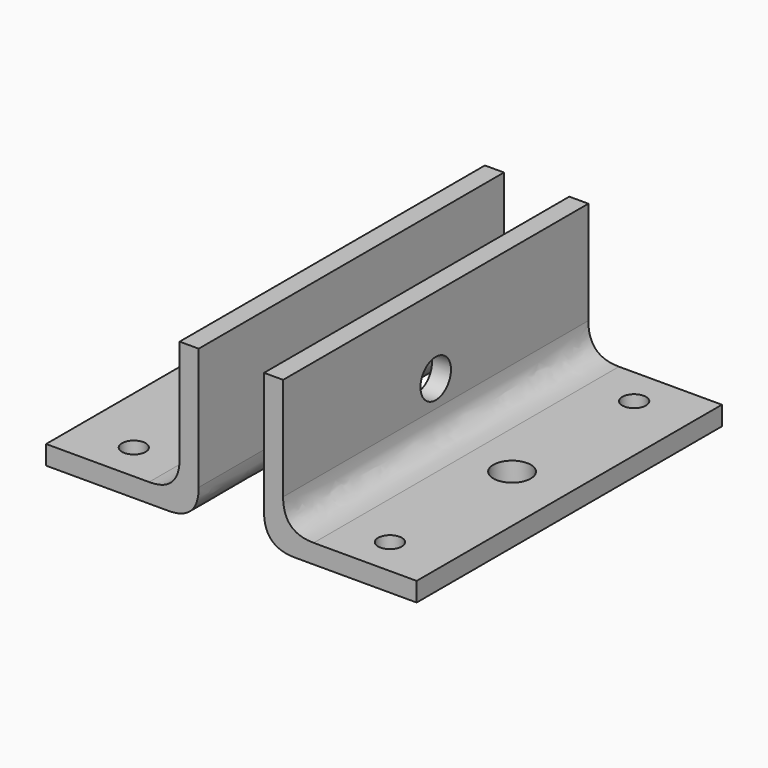
from build123d import *

# Parameters (mm, degrees)
F0_W           = 25.4
F0_H           = 63.5
F1_DEPTH       = 3.175
F2_W           = 3.175
F2_H           = 63.5
F3_DEPTH       = 22.225
F4_R           = 3.175
F5_DEPTH       = 3.175
F6_R           = 1.9685
F7_DEPTH       = 3.175
F8_R           = 1.9685
F9_DEPTH       = 3.175
F10_R          = 3.1115
F11_DEPTH      = 3.175
F12_W          = 25.4
F12_H          = 63.5
F13_DEPTH      = 3.175
F14_R          = 3.1115
F15_R          = 1.9685
F16_DEPTH      = 3.175
F17_W          = 3.175
F17_H          = 63.5
F18_DEPTH      = 22.225
F19_R          = 3.175
F20_DEPTH      = 3.175
F21_T1_DEPTH   = 63.5
F21_T3_DEPTH   = 88.9
F21_2_T1_DEPTH = 63.5
F21_2_T3_DEPTH = 88.9


# Not quite as in the source:
# - a fillet or chamfer that OpenCascade refuses, or shapes differently, is made with other operations: its cross-section is extruded or revolved along the edge and cut away or added


with BuildPart() as f1:
    # F0 (on Top) → F1 (new body)
    with BuildSketch(Plane.XY):
        with Locations((-29.1409659298, -4.4768862426)):
            Rectangle(F0_W, F0_H)
    extrude(amount=F1_DEPTH)

    # F2 (on face) → F3 (join)
    with BuildSketch(Plane.XY.offset(3.175)):
        with Locations((-18.0284659298, -4.4768862426)):
            Rectangle(F2_W, F2_H)
    extrude(amount=F3_DEPTH)

    # F4 (on face) → F5 (cut)
    with BuildSketch(Plane(origin=(-19.6159659298, 0, 0), x_dir=(0, -1, 0), z_dir=(-1, 0, 0))):
        with Locations((4.4768862426, 12.7)):
            Circle(F4_R)
    extrude(amount=-F5_DEPTH, mode=Mode.SUBTRACT)

    # F6 (on face) → F7 (cut)
    with BuildSketch(Plane.XY.offset(3.175)):
        with Locations((-32.3159659298, 20.9231137574)):
            Circle(F6_R)
    extrude(amount=-F7_DEPTH, mode=Mode.SUBTRACT)

    # F8 (on face) → F9 (cut)
    with BuildSketch(Plane.XY.offset(3.175)):
        with Locations((-32.3159659298, -29.8768862426)):
            Circle(F8_R)
    extrude(amount=-F9_DEPTH, mode=Mode.SUBTRACT)

    # F10 (on face) → F11 (cut)
    with BuildSketch(Plane.XY.offset(3.175)):
        with Locations((-32.3159659298, -4.4768862426)):
            Circle(F10_R)
    extrude(amount=-F11_DEPTH, mode=Mode.SUBTRACT)

    # F21: fillet of radius 5.08 on 2 edges, made by hand

    # F21_s2 → F21_t1 (join)
    with BuildSketch(Plane.XZ.offset(-27.2731137574)):
        with BuildLine():
            add(Edge.make_bspline(
                [(-19.6159659298, 8.255), (-19.6159659298, 3.175), (-24.6959659298, 3.175)],
                knots=[0, 0, 0, 1, 1, 1], degree=2, weights=[1, 1, 1]))
            Line((-24.6959659298, 3.175), (-19.6159659298, 3.175))
            Line((-19.6159659298, 3.175), (-19.6159659298, 8.255))
        make_face()
    extrude(amount=F21_T1_DEPTH)

    # F21_s4 → F21_t3 (cut)
    with BuildSketch(Plane.XZ.offset(-39.9731137574)):
        with BuildLine():
            add(Edge.make_bspline(
                [(-16.4409659298, 5.08), (-16.4409659298, 0), (-21.5209659298, 0)],
                knots=[0, 0, 0, 1, 1, 1], degree=2, weights=[1, 1, 1]))
            Line((-21.5209659298, 0), (-16.4409659298, 0))
            Line((-16.4409659298, 0), (-16.4409659298, 5.08))
        make_face()
    extrude(amount=F21_T3_DEPTH, mode=Mode.SUBTRACT)


with BuildPart() as f13:
    # F12 (on Top) → F13 (new body)
    with BuildSketch(Plane.XY):
        with Locations((7.1329429418, -4.4768862426)):
            Rectangle(F12_W, F12_H)
    extrude(amount=F13_DEPTH)

    # F14 (on face) + F15 (on face) → F16 (cut)
    with BuildSketch(Plane.XY.offset(3.175)):
        with Locations((10.3079429418, -4.4768862426)):
            Circle(F14_R)
    with BuildSketch(Plane.XY.offset(3.175)):
        with Locations((10.3079429418, 20.9231137574)):
            Circle(F15_R)
        with Locations((10.3079429418, -29.8768862426)):
            Circle(F15_R)
    extrude(amount=-F16_DEPTH, mode=Mode.SUBTRACT)

    # F17 (on face) → F18 (join)
    with BuildSketch(Plane.XY.offset(3.175)):
        with Locations((-3.9795570582, -4.4768862426)):
            Rectangle(F17_W, F17_H)
    extrude(amount=F18_DEPTH)

    # F19 (on face) → F20 (cut)
    with BuildSketch(Plane.YZ.offset(-2.3920570582)):
        with Locations((-4.4768862426, 12.7)):
            Circle(F19_R)
    extrude(amount=-F20_DEPTH, mode=Mode.SUBTRACT)

    # F21#2: fillet of radius 5.08 on 2 edges, made by hand

    # F21_2_s2 → F21_2_t1 (join)
    with BuildSketch(Plane.XZ.offset(-27.2731137574)):
        with BuildLine():
            add(Edge.make_bspline(
                [(2.6879429418, 3.175), (-2.3920570582, 3.175), (-2.3920570582, 8.255)],
                knots=[0, 0, 0, 1, 1, 1], degree=2, weights=[1, 1, 1]))
            Line((-2.3920570582, 8.255), (-2.3920570582, 3.175))
            Line((-2.3920570582, 3.175), (2.6879429418, 3.175))
        make_face()
    extrude(amount=F21_2_T1_DEPTH)

    # F21_2_s4 → F21_2_t3 (cut)
    with BuildSketch(Plane.XZ.offset(-39.9731137574)):
        with BuildLine():
            add(Edge.make_bspline(
                [(-5.5670570582, 5.08), (-5.5670570582, 0), (-0.4870570582, 0)],
                knots=[0, 0, 0, 1, 1, 1], degree=2, weights=[1, 1, 1]))
            Line((-0.4870570582, 0), (-5.5670570582, 0))
            Line((-5.5670570582, 0), (-5.5670570582, 5.08))
        make_face()
    extrude(amount=F21_2_T3_DEPTH, mode=Mode.SUBTRACT)


solid = Compound([f1.part, f13.part])
